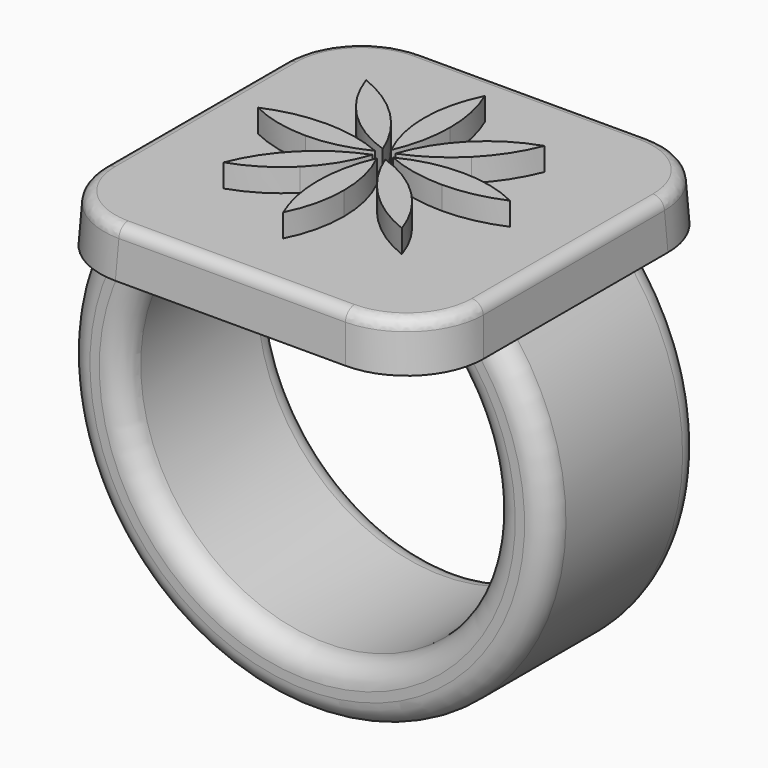
from build123d import *

# Parameters (mm, degrees)
F0_W      = 25.4
F0_H      = 25.4
F1_DEPTH  = 3.175
F1_TAPER  = 3
F3_W      = 5.08
F3_H      = 12.7
F6_R      = 5.08
F7_R      = 1.524
F8_R      = 0.762
F10_DEPTH = 1.524


# Not quite as in the source:
# - ends of sketch curves that miss each other by under 0.0002 mm in the source are joined


with BuildPart() as f1:
    # F0 (on Top) → F1 (new body)
    with BuildSketch(Plane.XY):
        Rectangle(F0_W, F0_H)
    extrude(amount=F1_DEPTH, taper=F1_TAPER)

    # F4: sweep along a path in F2
    with BuildLine(Plane.XZ) as f4_path:
        ThreePointArc((-10.16, 0), (0, -23.5582897328), (10.16, 0))
    # F3 (on face) → F4 (sweep)
    with BuildSketch(Plane(origin=(0, 0, 0), x_dir=(1, 0, 0), z_dir=(0, 0, -1))):
        with Locations((-10.16, 0)):
            Rectangle(F3_W, F3_H)
    sweep(path=f4_path.line)

    # F6
    f6_edges = [f1.edges().sort_by_distance(p)[0] for p in [
        (-12.616803, 12.616803, 1.5875),
        (-12.616803, -12.616803, 1.5875),
        (12.616803, -12.616803, 1.5875),
        (12.616803, 12.616803, 1.5875),
    ]]
    fillet(f6_edges, radius=F6_R)

    # F7
    f7_edges = [f1.edges().sort_by_distance(p)[0] for p in [
        (0, -6.35, -25.501344),
        (-1.743325, -6.35, -21.711017),
        (-1.743325, 6.35, -21.711017),
        (0, 6.35, -25.501344),
    ]]
    fillet(f7_edges, radius=F7_R)

    # F8
    f8_edges = [f1.edges().sort_by_distance(p)[0] for p in [
        (12.533605, 0, 3.175),
        (11.048589, -11.048589, 3.175),
        (11.048589, 11.048589, 3.175),
        (0, -12.533605, 3.175),
        (0, 12.533605, 3.175),
        (-11.048589, -11.048589, 3.175),
        (-11.048589, 11.048589, 3.175),
        (-12.533605, 0, 3.175),
    ]]
    fillet(f8_edges, radius=F8_R)

    # F9 (on face) → F10 (join)
    with BuildSketch(Plane.XY.offset(3.175)):
        with BuildLine():
            ThreePointArc((-3.8077433876, 2.5129958106), (-2.2363648369, 1.2700255802), (-0.4214138117, 0.4214041575))
            ThreePointArc((-0.4214138117, 0.4214041575), (-1.3351477858, 2.1876037686), (-2.5900078566, 3.7302233456))
            ThreePointArc((-2.5900078566, 3.7302233456), (-4.1334248315, 4.984630209), (-5.9002408115, 5.8978835339))
            ThreePointArc((-5.9002408115, 5.8978835339), (-5.0511449244, 4.0835594737), (-3.8077433876, 2.5129958106))
        make_face()
        with BuildLine():
            ThreePointArc((-0.9155427616, 4.4694347941), (-0.6833212656, 2.4793847644), (-1.9106e-05, 0.5959506396))
            ThreePointArc((-1.9106e-05, 0.5959506396), (0.6027711391, 2.4909604876), (0.8062465423, 4.4690791999))
            ThreePointArc((0.8062465423, 4.4690791999), (0.6018941572, 6.4474337167), (-0.0016602711, 8.3425243592))
            ThreePointArc((-0.0016602711, 8.3425243592), (-0.6841876238, 6.4592135153), (-0.9155427616, 4.4694347941))
        make_face()
        with BuildLine():
            ThreePointArc((2.5129831047, 3.8077560876), (1.2700048982, 2.2363724755), (0.4213787575, 0.4214138117))
            ThreePointArc((0.4213787575, 0.4214138117), (2.1875938836, 1.3351413072), (3.7302233456, 2.5900078566))
            ThreePointArc((3.7302233456, 2.5900078566), (4.984630209, 4.1334248315), (5.8978835339, 5.9002408115))
            ThreePointArc((5.8978835339, 5.9002408115), (4.0835594737, 5.0511449244), (2.5129831047, 3.8077560876))
        make_face()
        with BuildLine():
            ThreePointArc((4.4694347941, 0.9155427616), (2.4793737115, 0.6833186532), (0.5959303259, 8.9412e-06))
            ThreePointArc((0.5959303259, 8.9412e-06), (2.4909366547, -0.6027661778), (4.4690537999, -0.8062465482))
            ThreePointArc((4.4690537999, -0.8062465482), (6.4474197136, -0.6018917801), (8.3425203043, 0.0016695744))
            ThreePointArc((8.3425203043, 0.0016695744), (6.4592115314, 0.6841820987), (4.4694347941, 0.9155427616))
        make_face()
        with BuildLine():
            ThreePointArc((3.8077560876, -2.5129831047), (2.2363622238, -1.2699985662), (0.4213909469, -0.4213711439))
            ThreePointArc((0.4213909469, -0.4213711439), (1.3351159072, -2.1875938836), (2.5899824566, -3.7302233456))
            ThreePointArc((2.5899824566, -3.7302233456), (4.1334074282, -4.9846188126), (5.9002188082, -5.8978748887))
            ThreePointArc((5.9002188082, -5.8978748887), (5.0511428128, -4.0835560578), (3.8077560876, -2.5129831047))
        make_face()
        with BuildLine():
            ThreePointArc((0.9155173616, -4.4694348001), (0.6832945611, -2.4793792452), (-1.13725e-05, -0.5959404907))
            ThreePointArc((-1.13725e-05, -0.5959404907), (-0.6027905445, -2.4909316905), (-0.8062719482, -4.4690537999))
            ThreePointArc((-0.8062719482, -4.4690537999), (-0.601916144, -6.447424681), (0.0016482293, -8.3425296076))
            ThreePointArc((0.0016482293, -8.3425296076), (0.6841820987, -6.4592115314), (0.9155173616, -4.4694348001))
        make_face()
        with BuildLine():
            ThreePointArc((-2.5129958106, -3.8077433876), (-1.2700192482, -2.2363545852), (-0.4213965439, -0.4213909469))
            ThreePointArc((-0.4213965439, -0.4213909469), (-2.1876037686, -1.3351223858), (-3.7302233456, -2.5899824566))
            ThreePointArc((-3.7302233456, -2.5899824566), (-4.9846188126, -4.1334074282), (-5.8978748887, -5.9002188082))
            ThreePointArc((-5.8978748887, -5.9002188082), (-4.0835560578, -5.0511428128), (-2.5129958106, -3.8077433876))
        make_face()
        with BuildLine():
            ThreePointArc((-4.4694348001, -0.9155173616), (-2.4793902981, -0.6832971735), (-0.5959608043, 1.2077e-06))
            ThreePointArc((-0.5959608043, 1.2077e-06), (-2.4909555235, 0.6027955057), (-4.4690791999, 0.8062719423))
            ThreePointArc((-4.4690791999, 0.8062719423), (-6.4474386841, 0.6019185211), (-8.3425336625, -0.0016389259))
            ThreePointArc((-8.3425336625, -0.0016389259), (-6.4592135153, -0.6841876238), (-4.4694348001, -0.9155173616))
        make_face()
    extrude(amount=F10_DEPTH)


solid = f1.part
